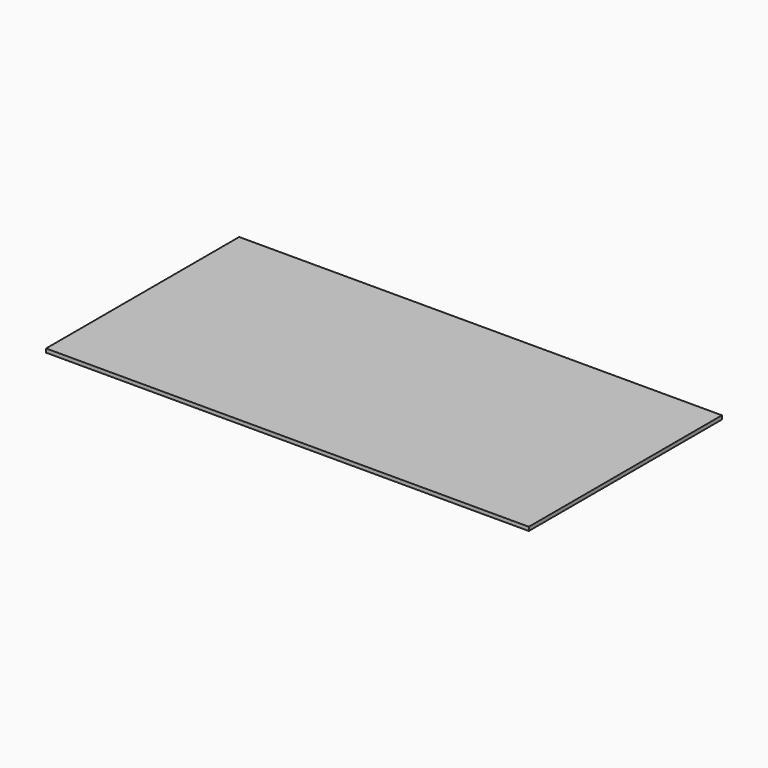
from build123d import *

# Parameters (mm, degrees)
F1_W     = 2438.4
F1_H     = 1219.2
F2_DEPTH = 19.05


# Not quite as in the source:
# - a variable given as a bare number and used for a length is read in inches; the dataset says mm whatever the document's units were


with BuildPart() as f2:
    # F1 (on Top) → F2 (new body)
    with BuildSketch(Plane.XY):
        Rectangle(F1_W, F1_H)
    extrude(amount=F2_DEPTH)


solid = f2.part
